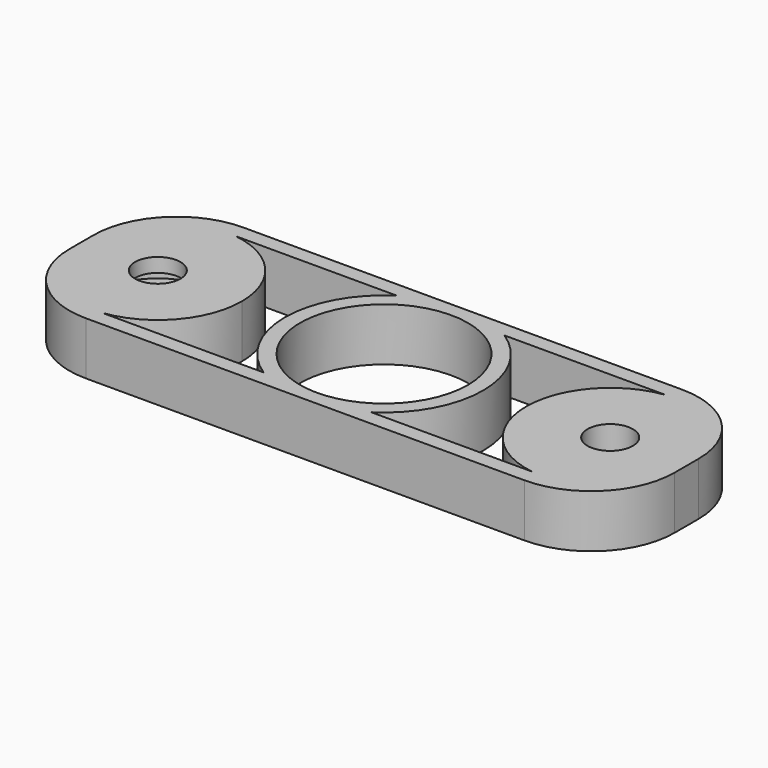
from build123d import *

# Parameters (mm, degrees)
F0_R      = 11.1
F1_DEPTH  = 3.5
F2_R      = 8.1
F4_DEPTH  = 1.65
F6_DEPTH  = 7.001
F7_R      = 3
F8_DEPTH  = 7.001
F9_R      = 3.875
F9_R_2    = 3
F10_DEPTH = 7


# Not quite as in the source:
# - a pattern or mirror of a feature is missing from the dataset's text; its kind, count and spacing are read off the source's solid


with BuildPart() as f1:
    # F0 (on Top) → F1 (new body, symmetric)
    with BuildSketch(Plane.XY):
        with BuildLine():
            ThreePointArc((40, 2), (36.7781745931, 9.7781745931), (29, 13))
            Line((29, 13), (-29, 13))
            ThreePointArc((-29, 13), (-36.7781745931, 9.7781745931), (-40, 2))
            Line((-40, 2), (-40, -2))
            ThreePointArc((-40, -2), (-36.7781745931, -9.7781745931), (-29, -13))
            Line((-29, -13), (29, -13))
            ThreePointArc((29, -13), (36.7781745931, -9.7781745931), (40, -2))
            Line((40, -2), (40, 2))
        make_face()
        Circle(F0_R, mode=Mode.SUBTRACT)
    extrude(amount=F1_DEPTH, both=True)

    # F2 (on Top) → F4 (cut, symmetric)
    with BuildSketch(Plane.XY):
        with Locations((-29.9, 0)):
            Circle(F2_R)
    f4 = extrude(amount=F4_DEPTH, both=True, mode=Mode.SUBTRACT)

    # F4_copies: F4 across plane
    add(f4.mirror(Plane(origin=(0, 0, 0), x_dir=(0, 0, 1), z_dir=(1, 0, 0))), mode=Mode.SUBTRACT)

    # F5 (on face) → F6 (cut, through all)
    with BuildSketch(Plane.XY.offset(3.5)):
        with BuildLine():
            ThreePointArc((-7.1140705647, -11), (-13.1, 0), (-7.1140705647, 11))
            Line((-7.1140705647, 11), (-28.4133931253, 11))
            ThreePointArc((-28.4133931253, 11), (-21.542029663, 7.3044049618), (-18.8, 0))
            ThreePointArc((-18.8, 0), (-21.542029663, -7.3044049618), (-28.4133931253, -11))
            Line((-28.4133931253, -11), (-7.1140705647, -11))
        make_face()
    f6 = extrude(amount=-F6_DEPTH, mode=Mode.SUBTRACT)

    # F6_copies: F6 across plane
    add(f6.mirror(Plane(origin=(0, 0, 0), x_dir=(0, 0, 1), z_dir=(1, 0, 0))), mode=Mode.SUBTRACT)

    # F7 (on face) → F8 (cut, through all)
    with BuildSketch(Plane.XY.offset(3.5)):
        with Locations((29.9, 0)):
            Circle(F7_R)
        with Locations((-29.9, 0)):
            Circle(F7_R)
    extrude(amount=-F8_DEPTH, mode=Mode.SUBTRACT)

    # F9 (on face) → F10 (join, through all)
    with BuildSketch(Plane.XY.offset(3.5)):
        with Locations((29.9, 0)):
            Circle(F9_R)
        with Locations((29.9, 0)):
            Circle(F9_R_2, mode=Mode.SUBTRACT)
    extrude(amount=-F10_DEPTH)


solid = f1.part
